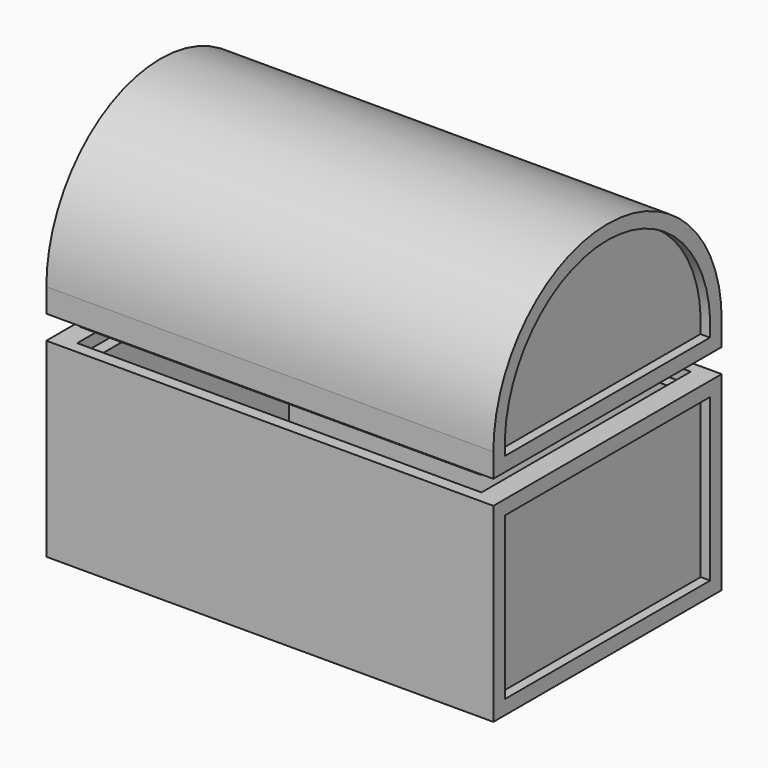
from build123d import *

# Parameters (mm, degrees)
F1_DEPTH  = 40
F2_W      = 60
F2_H      = 40
F3_DEPTH  = 5
F4_W      = 85
F4_H      = 54.9999991059
F4_W_2    = 80
F4_H_2    = 49.9999991059
F5_DEPTH  = 2.5
F8_DEPTH  = 40
F10_DEPTH = 5
F11_W     = 84.4
F11_H     = 54.4
F11_W_2   = 80
F11_H_2   = 50
F12_DEPTH = 2
F14_DEPTH = 2
F15_W     = 60
F15_H     = 40
F15_W_2   = 54
F15_H_2   = 34
F16_DEPTH = 2


# Not quite as in the source:
# - a pattern or mirror of a feature is missing from the dataset's text; its kind, count and spacing are read off the source's solid


with BuildPart() as f1:
    # F0 (on Right) → F1 (new body, symmetric)
    with BuildSketch(Plane.YZ):
        Polygon((-24.999999553, 0), (-30, 0), (-30, -40), (30, -40), (30, 0), (24.999999553, 0), (24.999999553, -34.999999553), (-24.999999553, -34.999999553), align=None)
    extrude(amount=F1_DEPTH, both=True)

    # F2 (on face) → F3 (join)
    with BuildSketch(Plane.YZ.offset(40)):
        with Locations((0, -20)):
            Rectangle(F2_W, F2_H)
    f3 = extrude(amount=F3_DEPTH)

    # F3_copies: F3 across plane
    add(f3.mirror(Plane(origin=(0, 0, 0), x_dir=(0, 0, -1), z_dir=(-1, 0, 0))))

    # F4 (on face) → F5 (cut)
    with BuildSketch(Plane.XY):
        Rectangle(F4_W, F4_H)
        Rectangle(F4_W_2, F4_H_2, mode=Mode.SUBTRACT)
    extrude(amount=-F5_DEPTH, mode=Mode.SUBTRACT)

    # F15 (on face) → F16 (join)
    with BuildSketch(Plane.YZ.offset(45)):
        with Locations((0, -20)):
            Rectangle(F15_W, F15_H)
        with Locations((0, -20)):
            Rectangle(F15_W_2, F15_H_2, mode=Mode.SUBTRACT)
    f16 = extrude(amount=F16_DEPTH)

    # F16_copies: F16 across plane
    add(f16.mirror(Plane(origin=(0, 0, 0), x_dir=(0, 0, -1), z_dir=(-1, 0, 0))))


with BuildPart() as f8:
    # F7 (on Right) → F8 (new body, symmetric)
    with BuildSketch(Plane.YZ):
        with BuildLine():
            Line((-30, 10), (-30, 5))
            Line((-30, 5), (-25, 5))
            Line((-25, 5), (-25, 10))
            ThreePointArc((-25, 10), (0, 35), (25, 10))
            Line((25, 10), (25, 5))
            Line((25, 5), (30, 5))
            Line((30, 5), (30, 10))
            ThreePointArc((30, 10), (0, 40), (-30, 10))
        make_face()
    extrude(amount=F8_DEPTH, both=True)

    # F9 (on face) → F10 (join)
    with BuildSketch(Plane.YZ.offset(40)):
        with BuildLine():
            Line((30, 5), (30, 10))
            ThreePointArc((30, 10), (0, 40), (-30, 10))
            Line((-30, 10), (-30, 5))
            Line((-30, 5), (30, 5))
        make_face()
    f10 = extrude(amount=F10_DEPTH)

    # F10_copies: F10 across plane
    add(f10.mirror(Plane(origin=(0, 0, 0), x_dir=(0, 0, -1), z_dir=(-1, 0, 0))))

    # F11 (on face) → F12 (join)
    with BuildSketch(Plane(origin=(0, 0, 5), x_dir=(1, 0, 0), z_dir=(0, 0, -1))):
        Rectangle(F11_W, F11_H)
        Rectangle(F11_W_2, F11_H_2, mode=Mode.SUBTRACT)
    extrude(amount=F12_DEPTH)

    # F13 (on face) → F14 (join)
    with BuildSketch(Plane.YZ.offset(45)):
        with BuildLine():
            ThreePointArc((30, 10), (0, 40), (-30, 10))
            Line((-30, 10), (-30, 5))
            Line((-30, 5), (30, 5))
            Line((30, 5), (30, 10))
        make_face()
        with BuildLine():
            ThreePointArc((-26.9258240357, 8), (0, 37), (26.9258240357, 8))
            Line((26.9258240357, 8), (-26.9258240357, 8))
        make_face(mode=Mode.SUBTRACT)
    f14 = extrude(amount=F14_DEPTH)

    # F14_copies: F14 across plane
    add(f14.mirror(Plane(origin=(0, 0, 0), x_dir=(0, 0, -1), z_dir=(-1, 0, 0))))


solid = Compound([f1.part, f8.part])
